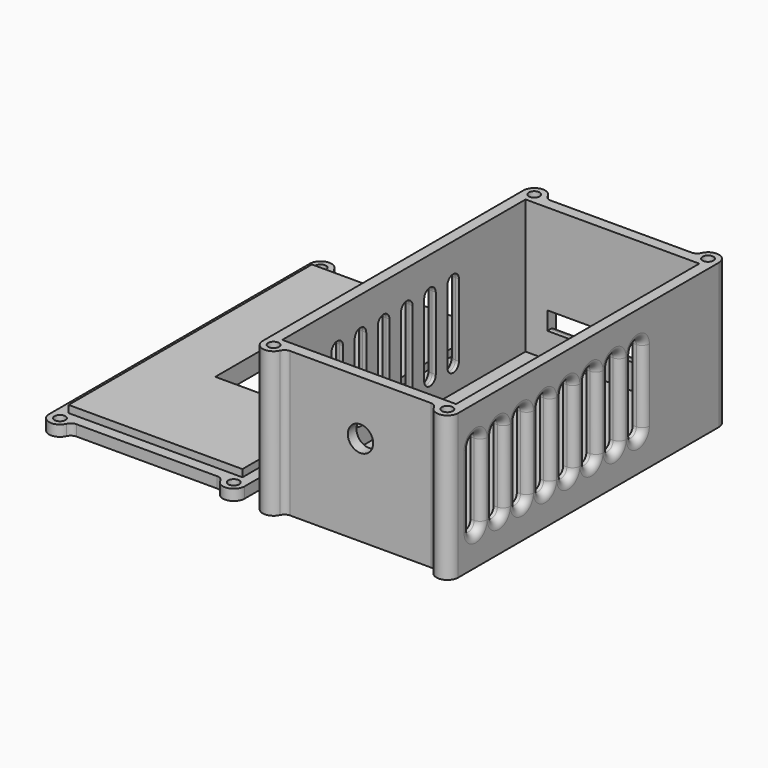
from build123d import *

# Parameters (mm, degrees)
F0_W      = 5
F0_H      = 1
F1_DEPTH  = 1
F0_R      = 1.5
F0_W_2    = 48
F0_H_2    = 84
F2_DEPTH  = 3
F0_W_3    = 15
F0_H_3    = 20
F3_DEPTH  = 5
F4_DEPTH  = 40
F5_W      = 36
F5_H      = 5
F6_DEPTH  = 5
F8_R      = 3.5
F9_DEPTH  = 15
F11_DEPTH = 60
F12_R     = 1.99999
F12_2_R   = 1.99999


# Not quite as in the source:
# - a fillet or chamfer is up to 0.001 mm smaller than in the source, because OpenCascade refuses the exact size


with BuildPart() as f1:
    # F0 (on Top) → F1 (new body)
    with BuildSketch(Plane.XY):
        with Locations((-2.5, -0.5)):
            Rectangle(F0_W, F0_H)
    extrude(amount=F1_DEPTH)

    # F0 (on Top) → F2 (join)
    with BuildSketch(Plane.XY):
        with BuildLine():
            Line((-5, -1), (-5, 0))
            ThreePointArc((-5, 0), (-8, 3), (-11, 0))
            Line((-11, 0), (-53, 0))
            ThreePointArc((-53, 0), (-56, 3), (-59, 0))
            Line((-59, 0), (-59, -90))
            ThreePointArc((-59, -90), (-56, -93), (-53, -90))
            Line((-53, -90), (-11, -90))
            ThreePointArc((-11, -90), (-8, -93), (-5, -90))
            Line((-5, -90), (-5, -1))
        make_face()
        with Locations((-56, -90)):
            Circle(F0_R, mode=Mode.SUBTRACT)
        with Locations((-8, -90)):
            Circle(F0_R, mode=Mode.SUBTRACT)
        with Locations((-32, -45)):
            Rectangle(F0_W_2, F0_H_2, mode=Mode.SUBTRACT)
        with Locations((-56, 0)):
            Circle(F0_R, mode=Mode.SUBTRACT)
        with Locations((-8, 0)):
            Circle(F0_R, mode=Mode.SUBTRACT)
    extrude(amount=F2_DEPTH)

    # F0 (on Top) → F3 (join)
    with BuildSketch(Plane.XY):
        with Locations((-32, -45)):
            Rectangle(F0_W_2, F0_H_2)
        with Locations((-32, -47)):
            Rectangle(F0_W_3, F0_H_3, mode=Mode.SUBTRACT)
    extrude(amount=F3_DEPTH)

    # F12#2 (radius 2 in the source; OpenCascade refuses exactly that, so slightly less here)
    f12_2_edges = [f1.edges().sort_by_distance(p)[0] for p in [
        (-53, 0, 1.5),
        (-11, 0, 1.5),
        (-11, -90, 1.5),
        (-53, -90, 1.5),
    ]]
    fillet(f12_2_edges, radius=F12_2_R)


with BuildPart() as f2:
    # F0 (on Top) → F2, piece 2 (new body)
    with BuildSketch(Plane.XY):
        with Locations((27, -45)):
            Rectangle(F0_W_2, F0_H_2)
    extrude(amount=F2_DEPTH)


with BuildPart() as f4:
    # F0 (on Top) → F4 (new body)
    with BuildSketch(Plane.XY):
        with BuildLine():
            ThreePointArc((6, 0), (3, 3), (0, 0))
            Line((0, 0), (0, -1))
            Line((0, -1), (0, -90))
            ThreePointArc((0, -90), (3, -93), (6, -90))
            Line((6, -90), (48, -90))
            ThreePointArc((48, -90), (51, -93), (54, -90))
            Line((54, -90), (54, 0))
            ThreePointArc((54, 0), (51, 3), (48, 0))
            Line((48, 0), (6, 0))
        make_face()
        with Locations((3, -90)):
            Circle(F0_R, mode=Mode.SUBTRACT)
        with Locations((51, -90)):
            Circle(F0_R, mode=Mode.SUBTRACT)
        with Locations((27, -45)):
            Rectangle(F0_W_2, F0_H_2, mode=Mode.SUBTRACT)
        with Locations((3, 0)):
            Circle(F0_R, mode=Mode.SUBTRACT)
        with Locations((51, 0)):
            Circle(F0_R, mode=Mode.SUBTRACT)
    extrude(amount=F4_DEPTH)

    # F5 (on Front) → F6 (cut)
    with BuildSketch(Plane.XZ):
        with Locations((27, 12.5)):
            Rectangle(F5_W, F5_H)
    extrude(amount=F6_DEPTH, mode=Mode.SUBTRACT)

    # F8 (on offset) → F9 (cut)
    with BuildSketch(Plane.XZ.offset(100)):
        with Locations((27, 25)):
            Circle(F8_R)
    extrude(amount=-F9_DEPTH, mode=Mode.SUBTRACT)

    # F10 (on Right) → F11 (cut)
    with BuildSketch(Plane.YZ):
        with BuildLine():
            ThreePointArc((-82, 30), (-84, 32), (-86, 30))
            Line((-86, 30), (-86, 10))
            ThreePointArc((-86, 10), (-84, 8), (-82, 10))
            Line((-82, 10), (-82, 30))
        make_face()
        with BuildLine():
            ThreePointArc((-74, 30), (-76, 32), (-78, 30))
            Line((-78, 30), (-78, 10))
            ThreePointArc((-78, 10), (-76, 8), (-74, 10))
            Line((-74, 10), (-74, 30))
        make_face()
        with BuildLine():
            Line((-66, 10), (-66, 30))
            ThreePointArc((-66, 30), (-68, 32), (-70, 30))
            Line((-70, 30), (-70, 10))
            ThreePointArc((-70, 10), (-68, 8), (-66, 10))
        make_face()
        with BuildLine():
            ThreePointArc((-62, 10), (-60, 8), (-58, 10))
            Line((-58, 10), (-58, 30))
            ThreePointArc((-58, 30), (-60, 32), (-62, 30))
            Line((-62, 30), (-62, 10))
        make_face()
        with BuildLine():
            Line((-50, 10), (-50, 30))
            ThreePointArc((-50, 30), (-52, 32), (-54, 30))
            Line((-54, 30), (-54, 10))
            ThreePointArc((-54, 10), (-52, 8), (-50, 10))
        make_face()
        with BuildLine():
            ThreePointArc((-42, 30), (-44, 32), (-46, 30))
            Line((-46, 30), (-46, 10))
            ThreePointArc((-46, 10), (-44, 8), (-42, 10))
            Line((-42, 10), (-42, 30))
        make_face()
        with BuildLine():
            Line((-34, 10), (-34, 30))
            ThreePointArc((-34, 30), (-36, 32), (-38, 30))
            Line((-38, 30), (-38, 10))
            ThreePointArc((-38, 10), (-36, 8), (-34, 10))
        make_face()
        with BuildLine():
            ThreePointArc((-26, 30), (-28, 32), (-30, 30))
            Line((-30, 30), (-30, 10))
            ThreePointArc((-30, 10), (-28, 8), (-26, 10))
            Line((-26, 10), (-26, 30))
        make_face()
    extrude(amount=F11_DEPTH, mode=Mode.SUBTRACT)

    # F12 (radius 2 in the source; OpenCascade refuses exactly that, so slightly less here)
    f12_edges = [f4.edges().sort_by_distance(p)[0] for p in [
        (48, -90, 20),
        (6, -90, 20),
        (54, -82, 20),
        (54, -74, 20),
        (54, -66, 20),
        (54, -58, 20),
        (54, -50, 20),
        (54, -42, 20),
        (54, -34, 20),
        (54, -26, 20),
        (0, -86, 20),
        (0, -78, 20),
        (0, -70, 20),
        (0, -58, 20),
        (0, -50, 20),
        (0, -42, 20),
        (0, -34, 20),
        (0, -26, 20),
        (48, 0, 20),
        (27, 0, 10),
        (27, 0, 15),
        (6, 0, 20),
    ]]
    fillet(f12_edges, radius=F12_R)


solid = Compound([f1.part, f2.part, f4.part])
